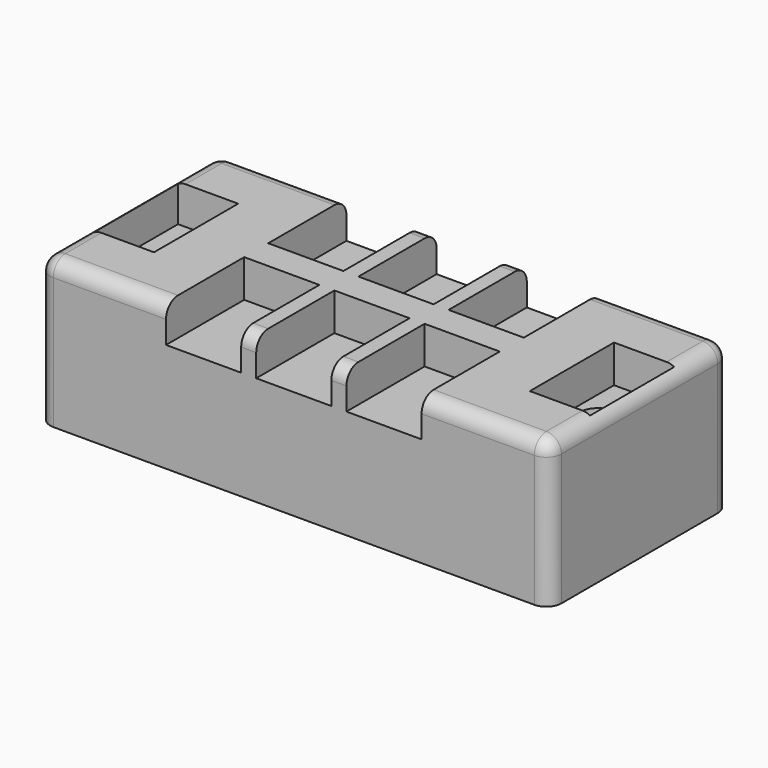
from build123d import *

# Parameters (mm, degrees)
F0_W         = 68
F0_H         = 30
F1_DEPTH     = 19.5
F2_R         = 2.5
F3_DEPTH     = 19.5
F4_W         = 10
F4_H         = 13
F4_W_2       = 8
F4_H_2       = 14
F5_DEPTH     = 5
F6_T1_DEPTH  = 20
F6_T3_DEPTH  = 26
F6_T5_DEPTH  = 20
F6_T7_DEPTH  = 12
F6_T9_DEPTH  = 12
F6_T11_DEPTH = 22.5
F6_S15_W     = 2
F6_S15_H     = 2
F6_T16_DEPTH = 2
F6_S21_W     = 2
F6_S21_H     = 2
F6_T22_DEPTH = 2
F6_S27_W     = 2
F6_S27_H     = 2
F6_T28_DEPTH = 2
F6_S33_W     = 2
F6_S33_H     = 2
F6_T34_DEPTH = 2


# Not quite as in the source:
# - a fillet or chamfer that OpenCascade refuses, or shapes differently, is made with other operations: its cross-section is extruded or revolved along the edge and cut away or added


with BuildPart() as f1:
    # F0 (on Top) → F1 (new body)
    with BuildSketch(Plane.XY):
        Rectangle(F0_W, F0_H)
    extrude(amount=F1_DEPTH)

    # F2 (on face) → F3 (cut, through all)
    with BuildSketch(Plane.XY.offset(19.5)):
        with Locations((-28.5, 0)):
            Circle(F2_R)
        with Locations((28.5, 0)):
            Circle(F2_R)
    extrude(amount=-F3_DEPTH, mode=Mode.SUBTRACT)

    # F4 (on face) → F5 (cut)
    with BuildSketch(Plane.XY.offset(19.5)):
        with Locations((0, 8.5)):
            Rectangle(F4_W, F4_H)
        with Locations((12, 8.5)):
            Rectangle(F4_W, F4_H)
        with Locations((-12, 8.5)):
            Rectangle(F4_W, F4_H)
        with Locations((-12, -8.5)):
            Rectangle(F4_W, F4_H)
        with Locations((0, -8.5)):
            Rectangle(F4_W, F4_H)
        with Locations((12, -8.5)):
            Rectangle(F4_W, F4_H)
        with Locations((29, 0)):
            Rectangle(F4_W_2, F4_H_2)
        with Locations((-29, 0)):
            Rectangle(F4_W_2, F4_H_2)
    extrude(amount=-F5_DEPTH, mode=Mode.SUBTRACT)

    # F6: fillet of radius 2 on 14 edges, made by hand

    # F6_s2 → F6_t1 (cut)
    with BuildSketch(Plane.YZ.offset(-32)):
        with BuildLine():
            ThreePointArc((-15, 17.5), (-14.4142135624, 18.9142135624), (-13, 19.5))
            Line((-13, 19.5), (-15, 19.5))
            Line((-15, 19.5), (-15, 17.5))
        make_face()
        with BuildLine():
            ThreePointArc((13, 19.5), (14.4142135624, 18.9142135624), (15, 17.5))
            Line((15, 17.5), (15, 19.5))
            Line((15, 19.5), (13, 19.5))
        make_face()
    extrude(amount=F6_T1_DEPTH, mode=Mode.SUBTRACT)

    # F6_s4 → F6_t3 (cut)
    with BuildSketch(Plane.XZ.offset(-13)):
        with BuildLine():
            ThreePointArc((-32, 19.5), (-33.4142135624, 18.9142135624), (-34, 17.5))
            Line((-34, 17.5), (-34, 19.5))
            Line((-34, 19.5), (-32, 19.5))
        make_face()
        with BuildLine():
            ThreePointArc((34, 17.5), (33.4142135624, 18.9142135624), (32, 19.5))
            Line((32, 19.5), (34, 19.5))
            Line((34, 19.5), (34, 17.5))
        make_face()
    extrude(amount=F6_T3_DEPTH, mode=Mode.SUBTRACT)

    # F6_s6 → F6_t5 (cut)
    with BuildSketch(Plane.YZ.offset(12)):
        with BuildLine():
            ThreePointArc((-15, 17.5), (-14.4142135624, 18.9142135624), (-13, 19.5))
            Line((-13, 19.5), (-15, 19.5))
            Line((-15, 19.5), (-15, 17.5))
        make_face()
        with BuildLine():
            ThreePointArc((13, 19.5), (14.4142135624, 18.9142135624), (15, 17.5))
            Line((15, 17.5), (15, 19.5))
            Line((15, 19.5), (13, 19.5))
        make_face()
    extrude(amount=F6_T5_DEPTH, mode=Mode.SUBTRACT)

    # F6_s8 → F6_t7 (cut)
    with BuildSketch(Plane.YZ):
        with BuildLine():
            ThreePointArc((-15, 17.5), (-14.4142135624, 18.9142135624), (-13, 19.5))
            Line((-13, 19.5), (-15, 19.5))
            Line((-15, 19.5), (-15, 17.5))
        make_face()
        with BuildLine():
            ThreePointArc((13, 19.5), (14.4142135624, 18.9142135624), (15, 17.5))
            Line((15, 17.5), (15, 19.5))
            Line((15, 19.5), (13, 19.5))
        make_face()
    extrude(amount=F6_T7_DEPTH, mode=Mode.SUBTRACT)

    # F6_s10 → F6_t9 (cut)
    with BuildSketch(Plane.YZ.offset(-12)):
        with BuildLine():
            ThreePointArc((-15, 17.5), (-14.4142135624, 18.9142135624), (-13, 19.5))
            Line((-13, 19.5), (-15, 19.5))
            Line((-15, 19.5), (-15, 17.5))
        make_face()
        with BuildLine():
            ThreePointArc((13, 19.5), (14.4142135624, 18.9142135624), (15, 17.5))
            Line((15, 17.5), (15, 19.5))
            Line((15, 19.5), (13, 19.5))
        make_face()
    extrude(amount=F6_T9_DEPTH, mode=Mode.SUBTRACT)

    # F6_s12 → F6_t11 (cut)
    with BuildSketch(Plane.XY.offset(-5)):
        with BuildLine():
            ThreePointArc((-32, -15), (-33.4142135624, -14.4142135624), (-34, -13))
            Line((-34, -13), (-34, -15))
            Line((-34, -15), (-32, -15))
        make_face()
        with BuildLine():
            ThreePointArc((-34, 13), (-33.4142135624, 14.4142135624), (-32, 15))
            Line((-32, 15), (-34, 15))
            Line((-34, 15), (-34, 13))
        make_face()
        with BuildLine():
            ThreePointArc((34, 13), (33.4142135624, 14.4142135624), (32, 15))
            Line((32, 15), (34, 15))
            Line((34, 15), (34, 13))
        make_face()
        with BuildLine():
            ThreePointArc((32, -15), (33.4142135624, -14.4142135624), (34, -13))
            Line((34, -13), (34, -15))
            Line((34, -15), (32, -15))
        make_face()
    extrude(amount=F6_T11_DEPTH, mode=Mode.SUBTRACT)


with BuildPart() as f6_tool14:
    # F6_s15 → F6_t16 (new body)
    with BuildSketch(Plane.XZ.offset(13)):
        with Locations((-33, 18.5)):
            Rectangle(F6_S15_W, F6_S15_H)
    extrude(amount=F6_T16_DEPTH)

    # F6_s17 → F6_t18 (revolve, cut)
    with BuildSketch(Plane(origin=(-32, -13, 17.5), x_dir=(0.7071067812, 0, -0.7071067812), z_dir=(-0.7071067812, 0, -0.7071067812))):
        with BuildLine():
            ThreePointArc((0, -2), (2, 0), (0, 2))
            Line((0, 2), (0, -2))
        make_face()
    revolve(axis=Axis((-32, -13, 17.5), (0, -1, 0)), mode=Mode.SUBTRACT)


with BuildPart() as f1_1:
    add(f1.part)

    # F6_t13: cut F6_tool14
    add(f6_tool14.part, mode=Mode.SUBTRACT)


with BuildPart() as f6_tool20:
    # F6_s21 → F6_t22 (new body)
    with BuildSketch(Plane.XY.offset(17.5)):
        with Locations((-33, 14)):
            Rectangle(F6_S21_W, F6_S21_H)
    extrude(amount=F6_T22_DEPTH)

    # F6_s23 → F6_t24 (revolve, cut)
    with BuildSketch(Plane(origin=(-32, 13, 17.5), x_dir=(0.7071067812, -0.7071067812, 0), z_dir=(-0.7071067812, -0.7071067812, 0))):
        with BuildLine():
            ThreePointArc((0, -2), (2, 0), (0, 2))
            Line((0, 2), (0, -2))
        make_face()
    revolve(axis=Axis((-32, 13, 17.5), (0, 0, 1)), mode=Mode.SUBTRACT)


with BuildPart() as f1_2:
    add(f1_1.part)

    # F6_t19: cut F6_tool20
    add(f6_tool20.part, mode=Mode.SUBTRACT)


with BuildPart() as f6_tool26:
    # F6_s27 → F6_t28 (new body)
    with BuildSketch(Plane.XZ.offset(13)):
        with Locations((33, 18.5)):
            Rectangle(F6_S27_W, F6_S27_H)
    extrude(amount=F6_T28_DEPTH)

    # F6_s29 → F6_t30 (revolve, cut)
    with BuildSketch(Plane(origin=(32, -13, 17.5), x_dir=(-0.7071067812, 0, -0.7071067812), z_dir=(-0.7071067812, 0, 0.7071067812))):
        with BuildLine():
            ThreePointArc((0, -2), (2, 0), (0, 2))
            Line((0, 2), (0, -2))
        make_face()
    revolve(axis=Axis((32, -13, 17.5), (0, -1, 0)), mode=Mode.SUBTRACT)


with BuildPart() as f1_3:
    add(f1_2.part)

    # F6_t25: cut F6_tool26
    add(f6_tool26.part, mode=Mode.SUBTRACT)


with BuildPart() as f6_tool32:
    # F6_s33 → F6_t34 (new body)
    with BuildSketch(Plane.YZ.offset(32)):
        with Locations((14, 18.5)):
            Rectangle(F6_S33_W, F6_S33_H)
    extrude(amount=F6_T34_DEPTH)

    # F6_s35 → F6_t36 (revolve, cut)
    with BuildSketch(Plane(origin=(32, 13, 17.5), x_dir=(0, -0.7071067812, -0.7071067812), z_dir=(0, -0.7071067812, 0.7071067812))):
        with BuildLine():
            ThreePointArc((0, -2), (2, 0), (0, 2))
            Line((0, 2), (0, -2))
        make_face()
    revolve(axis=Axis((32, 13, 17.5), (1, 0, 0)), mode=Mode.SUBTRACT)


with BuildPart() as f1_4:
    add(f1_3.part)

    # F6_t31: cut F6_tool32
    add(f6_tool32.part, mode=Mode.SUBTRACT)


solid = f1_4.part
